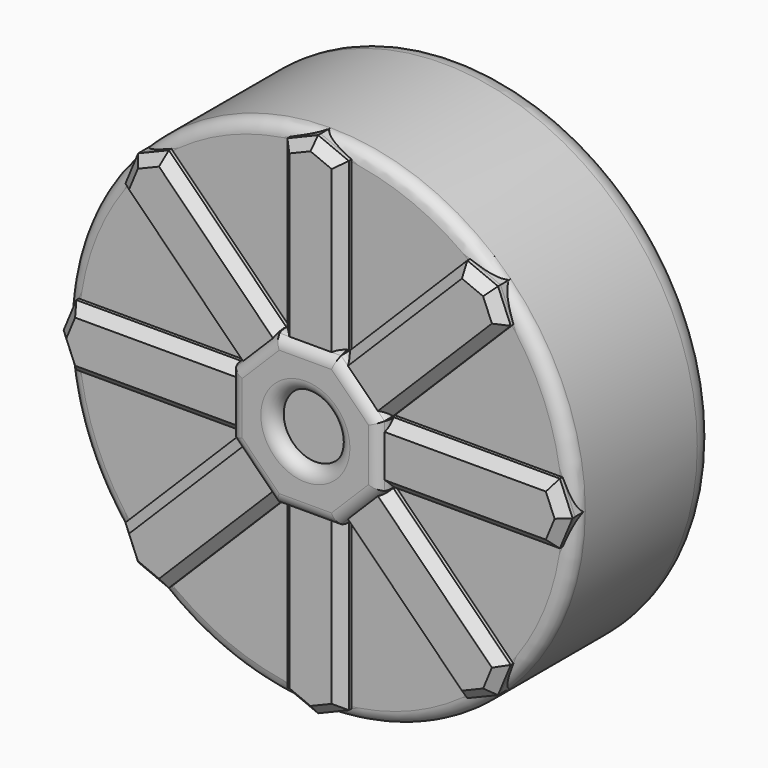
from build123d import *

# Parameters (mm, degrees)
F0_R           = 20
F1_DEPTH       = 14
F3_DEPTH       = 1
F5_DEPTH       = 0.5
F6_R           = 2.5
F7_DEPTH       = 1
F8_T4_ANGLE    = 45
F8_T9_ANGLE    = 45
F8_T15_ANGLE   = 45
F8_T20_ANGLE   = 45
F8_T26_ANGLE   = 45
F8_T31_ANGLE   = 45
F8_T37_ANGLE   = 45
F8_T42_ANGLE   = 45
F8_T48_ANGLE   = 45
F8_T53_ANGLE   = 45
F8_T59_ANGLE   = 45
F8_T64_ANGLE   = 45
F8_T70_ANGLE   = 45
F8_T75_ANGLE   = 45
F8_T81_ANGLE   = 45
F8_T86_ANGLE   = 45
F9_T1_DEPTH    = 9.1585541437
F9_T3_DEPTH    = 9.1585541437
F9_T5_DEPTH    = 9.1585541437
F9_T7_DEPTH    = 9.1585541437
F9_T9_DEPTH    = 9.1585541437
F9_T11_DEPTH   = 9.1585541437
F10_T1_DEPTH   = 6.4706504117
F10_T3_DEPTH   = 6.4706504117
F10_T5_DEPTH   = 6.4706504117
F10_T7_DEPTH   = 6.4706504117
F10_T9_DEPTH   = 6.4706504117
F10_T11_DEPTH  = 6.4706504117
F10_T13_DEPTH  = 6.4706504117
F10_T15_DEPTH  = 6.4706504117
F10_T17_DEPTH  = 6.4706504117
F10_T19_DEPTH  = 6.4706504117
F10_T21_DEPTH  = 6.4706504117
F10_T23_DEPTH  = 6.4706504117
F10_T25_DEPTH  = 6.4706504117
F10_T27_DEPTH  = 6.4706504117
F10_T29_DEPTH  = 6.4706504117
F10_T31_DEPTH  = 6.4706504117
F10_T36_DEPTH  = 17.0290973572
F10_S38_R      = 0.9999999996
F10_T39_DEPTH  = 10
F10_T43_DEPTH  = 17.0290973572
F10_S45_R      = 0.9999999996
F10_T46_DEPTH  = 10
F10_T50_DEPTH  = 17.0290973572
F10_S52_R      = 0.9999999996
F10_T53_DEPTH  = 10
F10_T57_DEPTH  = 17.0290973572
F10_S59_R      = 0.9999999996
F10_T60_DEPTH  = 10
F10_T64_DEPTH  = 17.0290973572
F10_S66_R      = 0.9999999996
F10_T67_DEPTH  = 10
F10_T71_DEPTH  = 17.0290973572
F10_S73_R      = 0.9999999996
F10_T74_DEPTH  = 10
F10_T78_DEPTH  = 17.0290973572
F10_S80_R      = 0.9999999996
F10_T81_DEPTH  = 10
F10_T85_DEPTH  = 17.0290973572
F10_S87_R      = 0.9999999996
F10_T88_DEPTH  = 10
F10_T92_DEPTH  = 17.0290973572
F10_S94_R      = 0.9999999996
F10_T95_DEPTH  = 10
F10_T99_DEPTH  = 17.0290973572
F10_S101_R     = 0.9999999996
F10_T102_DEPTH = 10
F10_T106_DEPTH = 17.0290973572
F10_S108_R     = 0.9999999996
F10_T109_DEPTH = 10
F10_T113_DEPTH = 17.0290973572
F10_S115_R     = 0.9999999996
F10_T116_DEPTH = 10
F10_T120_DEPTH = 17.0290973572
F10_S122_R     = 0.9999999996
F10_T123_DEPTH = 10
F10_T127_DEPTH = 17.0290973572
F10_S129_R     = 0.9999999996
F10_T130_DEPTH = 10
F10_T134_DEPTH = 17.0290973572
F10_S136_R     = 0.9999999996
F10_T137_DEPTH = 10
F10_T141_DEPTH = 17.0290973572
F10_S143_R     = 0.9999999996
F10_T144_DEPTH = 10
F11_R          = 2


# Not quite as in the source:
# - a fillet or chamfer that OpenCascade refuses, or shapes differently, is made with other operations: its cross-section is extruded or revolved along the edge and cut away or added


with BuildPart() as f1:
    # F0 (on Front) → F1 (new body)
    with BuildSketch(Plane.XZ):
        Circle(F0_R)
    extrude(amount=F1_DEPTH)

    # F2 (on face) → F3 (join)
    with BuildSketch(Plane.XZ.offset(14)):
        Polygon((15.1421356237, 11.7279220614), (14.1421356237, 14.1421356237), (11.7279220614, 15.1421356237), (2.4142135624, 5.8284271247), (2.4142135624, 19), (0, 20), (-2.4142135624, 19), (-2.4142135624, 5.8284271247), (-11.7279220614, 15.1421356237), (-14.1421356237, 14.1421356237), (-15.1421356237, 11.7279220614), (-5.8284271247, 2.4142135624), (-19, 2.4142135624), (-20, 0), (-19, -2.4142135624), (-5.8284271247, -2.4142135624), (-15.1421356237, -11.7279220614), (-14.1421356237, -14.1421356237), (-11.7279220614, -15.1421356237), (-2.4142135624, -5.8284271247), (-2.4142135624, -19), (0, -20), (2.4142135624, -19), (2.4142135624, -5.8284271247), (11.7279220614, -15.1421356237), (14.1421356237, -14.1421356237), (15.1421356237, -11.7279220614), (5.8284271247, -2.4142135624), (19, -2.4142135624), (20, 0), (19, 2.4142135624), (5.8284271247, 2.4142135624), align=None)
    extrude(amount=F3_DEPTH)

    # F4 (on face) → F5 (join)
    with BuildSketch(Plane.XZ.offset(15)):
        Polygon((2.4142135624, 5.8284271247), (-2.4142135624, 5.8284271247), (-5.8284271247, 2.4142135624), (-5.8284271247, -2.4142135624), (-2.4142135624, -5.8284271247), (2.4142135624, -5.8284271247), (5.8284271247, -2.4142135624), (5.8284271247, 2.4142135624), align=None)
    extrude(amount=F5_DEPTH)

    # F6 (on face) → F7 (cut)
    with BuildSketch(Plane.XZ.offset(15.5)):
        Circle(F6_R)
    extrude(amount=-F7_DEPTH, mode=Mode.SUBTRACT)

    # F8: fillet of radius 1 on 8 edges, made by hand


with BuildPart() as f8_tool2:
    # F8_s3 → F8_t4 (revolve)
    with BuildSketch(Plane(origin=(0, 0, 0), x_dir=(0, 1, 0), z_dir=(0.7071067812, 0, 0.7071067812))):
        with BuildLine():
            ThreePointArc((-13, 20), (-13.7071067812, 19.7071067812), (-14, 19))
            Line((-14, 19), (-14, 20))
            Line((-14, 20), (-13, 20))
        make_face()
    revolve(axis=Axis((0, -14, 0), (0, -1, 0)), revolution_arc=F8_T4_ANGLE)

    split(bisect_by=Plane(origin=(-17.0710678119, 0, 7.0710678119), x_dir=(0, 1, 0), z_dir=(-0.9238795325, 0, 0.3826834324)), keep=Keep.TOP)


with BuildPart() as f1_1:
    add(f1.part)

    # F8_t1: cut F8_tool2
    add(f8_tool2.part, mode=Mode.SUBTRACT)


with BuildPart() as f8_tool7:
    # F8_s8 → F8_t9 (revolve)
    with BuildSketch(Plane(origin=(0, 0, 0), x_dir=(0, 1, 0), z_dir=(0.7071067812, 0, 0.7071067812))):
        with BuildLine():
            ThreePointArc((-13, 20), (-13.7071067812, 19.7071067812), (-14, 19))
            Line((-14, 19), (-14, 20))
            Line((-14, 20), (-13, 20))
        make_face()
    revolve(axis=Axis((0, -14, 0), (0, -1, 0)), revolution_arc=F8_T9_ANGLE)

    split(bisect_by=Plane(origin=(-1.7071067812, 0, -1.7071067812), x_dir=(0, 1, 0), z_dir=(-0.7071067812, 0, -0.7071067812)), keep=Keep.TOP)

    split(bisect_by=Plane.XY.offset(2.4142135624), keep=Keep.TOP)


with BuildPart() as f1_2:
    add(f1_1.part)

    # F8_t6: cut F8_tool7
    add(f8_tool7.part, mode=Mode.SUBTRACT)


with BuildPart() as f8_tool13:
    # F8_s14 → F8_t15 (revolve)
    with BuildSketch(Plane.XY):
        with BuildLine():
            ThreePointArc((-20, -13), (-19.7071067812, -13.7071067812), (-19, -14))
            Line((-19, -14), (-20, -14))
            Line((-20, -14), (-20, -13))
        make_face()
    revolve(axis=Axis((0, -14, 0), (0, -1, 0)), revolution_arc=F8_T15_ANGLE)

    split(bisect_by=Plane(origin=(-17.0710678119, 0, -7.0710678119), x_dir=(0, 1, 0), z_dir=(-0.9238795325, 0, -0.3826834324)), keep=Keep.TOP)


with BuildPart() as f1_3:
    add(f1_2.part)

    # F8_t12: cut F8_tool13
    add(f8_tool13.part, mode=Mode.SUBTRACT)


with BuildPart() as f8_tool18:
    # F8_s19 → F8_t20 (revolve)
    with BuildSketch(Plane.XY):
        with BuildLine():
            ThreePointArc((-20, -13), (-19.7071067812, -13.7071067812), (-19, -14))
            Line((-19, -14), (-20, -14))
            Line((-20, -14), (-20, -13))
        make_face()
    revolve(axis=Axis((0, -14, 0), (0, -1, 0)), revolution_arc=F8_T20_ANGLE)

    split(bisect_by=Plane.XY.offset(-2.4142135624), keep=Keep.BOTTOM)

    split(bisect_by=Plane(origin=(-1.7071067812, 0, 1.7071067812), x_dir=(0, 1, 0), z_dir=(-0.7071067812, 0, 0.7071067812)), keep=Keep.TOP)


with BuildPart() as f1_4:
    add(f1_3.part)

    # F8_t17: cut F8_tool18
    add(f8_tool18.part, mode=Mode.SUBTRACT)


with BuildPart() as f8_tool24:
    # F8_s25 → F8_t26 (revolve)
    with BuildSketch(Plane.YZ):
        with BuildLine():
            ThreePointArc((-13, 20), (-13.7071067812, 19.7071067812), (-14, 19))
            Line((-14, 19), (-14, 20))
            Line((-14, 20), (-13, 20))
        make_face()
    revolve(axis=Axis((0, -14, 0), (0, -1, 0)), revolution_arc=F8_T26_ANGLE)

    split(bisect_by=Plane(origin=(-7.0710678119, 0, 17.0710678119), x_dir=(0, 1, 0), z_dir=(-0.3826834324, 0, 0.9238795325)), keep=Keep.TOP)


with BuildPart() as f1_5:
    add(f1_4.part)

    # F8_t23: cut F8_tool24
    add(f8_tool24.part, mode=Mode.SUBTRACT)


with BuildPart() as f8_tool29:
    # F8_s30 → F8_t31 (revolve)
    with BuildSketch(Plane.YZ):
        with BuildLine():
            ThreePointArc((-13, 20), (-13.7071067812, 19.7071067812), (-14, 19))
            Line((-14, 19), (-14, 20))
            Line((-14, 20), (-13, 20))
        make_face()
    revolve(axis=Axis((0, -14, 0), (0, -1, 0)), revolution_arc=F8_T31_ANGLE)

    split(bisect_by=Plane.YZ.offset(-2.4142135624), keep=Keep.BOTTOM)

    split(bisect_by=Plane(origin=(1.7071067812, 0, 1.7071067812), x_dir=(0, 1, 0), z_dir=(0.7071067812, 0, 0.7071067812)), keep=Keep.TOP)


with BuildPart() as f1_6:
    add(f1_5.part)

    # F8_t28: cut F8_tool29
    add(f8_tool29.part, mode=Mode.SUBTRACT)


with BuildPart() as f8_tool35:
    # F8_s36 → F8_t37 (revolve)
    with BuildSketch(Plane(origin=(0, 0, 0), x_dir=(0, 1, 0), z_dir=(0.7071067812, 0, -0.7071067812))):
        with BuildLine():
            ThreePointArc((-13, 20), (-13.7071067812, 19.7071067812), (-14, 19))
            Line((-14, 19), (-14, 20))
            Line((-14, 20), (-13, 20))
        make_face()
    revolve(axis=Axis((0, -14, 0), (0, -1, 0)), revolution_arc=F8_T37_ANGLE)

    split(bisect_by=Plane(origin=(7.0710678119, 0, 17.0710678119), x_dir=(0, 1, 0), z_dir=(0.3826834324, 0, 0.9238795325)), keep=Keep.TOP)


with BuildPart() as f1_7:
    add(f1_6.part)

    # F8_t34: cut F8_tool35
    add(f8_tool35.part, mode=Mode.SUBTRACT)


with BuildPart() as f8_tool40:
    # F8_s41 → F8_t42 (revolve)
    with BuildSketch(Plane(origin=(0, 0, 0), x_dir=(0, 1, 0), z_dir=(0.7071067812, 0, -0.7071067812))):
        with BuildLine():
            ThreePointArc((-13, 20), (-13.7071067812, 19.7071067812), (-14, 19))
            Line((-14, 19), (-14, 20))
            Line((-14, 20), (-13, 20))
        make_face()
    revolve(axis=Axis((0, -14, 0), (0, -1, 0)), revolution_arc=F8_T42_ANGLE)

    split(bisect_by=Plane(origin=(-1.7071067812, 0, 1.7071067812), x_dir=(0, 1, 0), z_dir=(-0.7071067812, 0, 0.7071067812)), keep=Keep.TOP)

    split(bisect_by=Plane.YZ.offset(2.4142135624), keep=Keep.TOP)


with BuildPart() as f1_8:
    add(f1_7.part)

    # F8_t39: cut F8_tool40
    add(f8_tool40.part, mode=Mode.SUBTRACT)


with BuildPart() as f8_tool46:
    # F8_s47 → F8_t48 (revolve)
    with BuildSketch(Plane.XY):
        with BuildLine():
            ThreePointArc((20, -13), (19.7071067812, -13.7071067812), (19, -14))
            Line((19, -14), (20, -14))
            Line((20, -14), (20, -13))
        make_face()
    revolve(axis=Axis((0, -14, 0), (0, -1, 0)), revolution_arc=F8_T48_ANGLE)

    split(bisect_by=Plane(origin=(17.0710678119, 0, 7.0710678119), x_dir=(0, 1, 0), z_dir=(0.9238795325, 0, 0.3826834324)), keep=Keep.TOP)


with BuildPart() as f1_9:
    add(f1_8.part)

    # F8_t45: cut F8_tool46
    add(f8_tool46.part, mode=Mode.SUBTRACT)


with BuildPart() as f8_tool51:
    # F8_s52 → F8_t53 (revolve)
    with BuildSketch(Plane.XY):
        with BuildLine():
            ThreePointArc((20, -13), (19.7071067812, -13.7071067812), (19, -14))
            Line((19, -14), (20, -14))
            Line((20, -14), (20, -13))
        make_face()
    revolve(axis=Axis((0, -14, 0), (0, -1, 0)), revolution_arc=F8_T53_ANGLE)

    split(bisect_by=Plane.XY.offset(2.4142135624), keep=Keep.TOP)

    split(bisect_by=Plane(origin=(1.7071067812, 0, -1.7071067812), x_dir=(0, 1, 0), z_dir=(0.7071067812, 0, -0.7071067812)), keep=Keep.TOP)


with BuildPart() as f1_10:
    add(f1_9.part)

    # F8_t50: cut F8_tool51
    add(f8_tool51.part, mode=Mode.SUBTRACT)


with BuildPart() as f8_tool57:
    # F8_s58 → F8_t59 (revolve)
    with BuildSketch(Plane(origin=(0, 0, 0), x_dir=(0, 1, 0), z_dir=(-0.7071067812, 0, -0.7071067812))):
        with BuildLine():
            ThreePointArc((-13, 20), (-13.7071067812, 19.7071067812), (-14, 19))
            Line((-14, 19), (-14, 20))
            Line((-14, 20), (-13, 20))
        make_face()
    revolve(axis=Axis((0, -14, 0), (0, -1, 0)), revolution_arc=F8_T59_ANGLE)

    split(bisect_by=Plane(origin=(17.0710678119, 0, -7.0710678119), x_dir=(0, 1, 0), z_dir=(0.9238795325, 0, -0.3826834324)), keep=Keep.TOP)


with BuildPart() as f1_11:
    add(f1_10.part)

    # F8_t56: cut F8_tool57
    add(f8_tool57.part, mode=Mode.SUBTRACT)


with BuildPart() as f8_tool62:
    # F8_s63 → F8_t64 (revolve)
    with BuildSketch(Plane(origin=(0, 0, 0), x_dir=(0, 1, 0), z_dir=(-0.7071067812, 0, -0.7071067812))):
        with BuildLine():
            ThreePointArc((-13, 20), (-13.7071067812, 19.7071067812), (-14, 19))
            Line((-14, 19), (-14, 20))
            Line((-14, 20), (-13, 20))
        make_face()
    revolve(axis=Axis((0, -14, 0), (0, -1, 0)), revolution_arc=F8_T64_ANGLE)

    split(bisect_by=Plane(origin=(1.7071067812, 0, 1.7071067812), x_dir=(0, 1, 0), z_dir=(0.7071067812, 0, 0.7071067812)), keep=Keep.TOP)

    split(bisect_by=Plane.XY.offset(-2.4142135624), keep=Keep.BOTTOM)


with BuildPart() as f1_12:
    add(f1_11.part)

    # F8_t61: cut F8_tool62
    add(f8_tool62.part, mode=Mode.SUBTRACT)


with BuildPart() as f8_tool68:
    # F8_s69 → F8_t70 (revolve)
    with BuildSketch(Plane.YZ):
        with BuildLine():
            ThreePointArc((-13, -20), (-13.7071067812, -19.7071067812), (-14, -19))
            Line((-14, -19), (-14, -20))
            Line((-14, -20), (-13, -20))
        make_face()
    revolve(axis=Axis((0, -14, 0), (0, -1, 0)), revolution_arc=F8_T70_ANGLE)

    split(bisect_by=Plane(origin=(7.0710678119, 0, -17.0710678119), x_dir=(0, 1, 0), z_dir=(0.3826834324, 0, -0.9238795325)), keep=Keep.TOP)


with BuildPart() as f1_13:
    add(f1_12.part)

    # F8_t67: cut F8_tool68
    add(f8_tool68.part, mode=Mode.SUBTRACT)


with BuildPart() as f8_tool73:
    # F8_s74 → F8_t75 (revolve)
    with BuildSketch(Plane.YZ):
        with BuildLine():
            ThreePointArc((-13, -20), (-13.7071067812, -19.7071067812), (-14, -19))
            Line((-14, -19), (-14, -20))
            Line((-14, -20), (-13, -20))
        make_face()
    revolve(axis=Axis((0, -14, 0), (0, -1, 0)), revolution_arc=F8_T75_ANGLE)

    split(bisect_by=Plane.YZ.offset(2.4142135624), keep=Keep.TOP)

    split(bisect_by=Plane(origin=(-1.7071067812, 0, -1.7071067812), x_dir=(0, 1, 0), z_dir=(-0.7071067812, 0, -0.7071067812)), keep=Keep.TOP)


with BuildPart() as f1_14:
    add(f1_13.part)

    # F8_t72: cut F8_tool73
    add(f8_tool73.part, mode=Mode.SUBTRACT)


with BuildPart() as f8_tool79:
    # F8_s80 → F8_t81 (revolve)
    with BuildSketch(Plane(origin=(0, 0, 0), x_dir=(0, 1, 0), z_dir=(-0.7071067812, 0, 0.7071067812))):
        with BuildLine():
            ThreePointArc((-13, 20), (-13.7071067812, 19.7071067812), (-14, 19))
            Line((-14, 19), (-14, 20))
            Line((-14, 20), (-13, 20))
        make_face()
    revolve(axis=Axis((0, -14, 0), (0, -1, 0)), revolution_arc=F8_T81_ANGLE)

    split(bisect_by=Plane(origin=(-7.0710678119, 0, -17.0710678119), x_dir=(0, 1, 0), z_dir=(-0.3826834324, 0, -0.9238795325)), keep=Keep.TOP)


with BuildPart() as f1_15:
    add(f1_14.part)

    # F8_t78: cut F8_tool79
    add(f8_tool79.part, mode=Mode.SUBTRACT)


with BuildPart() as f8_tool84:
    # F8_s85 → F8_t86 (revolve)
    with BuildSketch(Plane(origin=(0, 0, 0), x_dir=(0, 1, 0), z_dir=(-0.7071067812, 0, 0.7071067812))):
        with BuildLine():
            ThreePointArc((-13, 20), (-13.7071067812, 19.7071067812), (-14, 19))
            Line((-14, 19), (-14, 20))
            Line((-14, 20), (-13, 20))
        make_face()
    revolve(axis=Axis((0, -14, 0), (0, -1, 0)), revolution_arc=F8_T86_ANGLE)

    split(bisect_by=Plane(origin=(1.7071067812, 0, -1.7071067812), x_dir=(0, 1, 0), z_dir=(0.7071067812, 0, -0.7071067812)), keep=Keep.TOP)

    split(bisect_by=Plane.YZ.offset(-2.4142135624), keep=Keep.BOTTOM)


with BuildPart() as f1_16:
    add(f1_15.part)

    # F8_t83: cut F8_tool84
    add(f8_tool84.part, mode=Mode.SUBTRACT)

    # F9: fillet of radius 1 on 9 edges, made by hand

    # F9_s2 → F9_t1 (cut)
    with BuildSketch(Plane.YZ.offset(-4.5792770718)):
        with BuildLine():
            ThreePointArc((-15.5, 4.962401721), (-15.3660254038, 5.462401721), (-15, 5.8284271247))
            Line((-15, 5.8284271247), (-15.5, 5.8284271247))
            Line((-15.5, 5.8284271247), (-15.5, 4.962401721))
        make_face()
        with BuildLine():
            ThreePointArc((-15.5, -4.962401721), (-15.3660254038, -5.462401721), (-15, -5.8284271247))
            Line((-15, -5.8284271247), (-15.5, -5.8284271247))
            Line((-15.5, -5.8284271247), (-15.5, -4.962401721))
        make_face()
    extrude(amount=F9_T1_DEPTH, mode=Mode.SUBTRACT)

    # F9_s4 → F9_t3 (cut)
    with BuildSketch(Plane(origin=(3.2380378704, 0, -3.2380378704), x_dir=(0, 1, 0), z_dir=(-0.7071067812, 0, 0.7071067812))):
        with BuildLine():
            ThreePointArc((-15.5, -4.962401721), (-15.3660254038, -5.462401721), (-15, -5.8284271247))
            Line((-15, -5.8284271247), (-15.5, -5.8284271247))
            Line((-15.5, -5.8284271247), (-15.5, -4.962401721))
        make_face()
    extrude(amount=F9_T3_DEPTH, mode=Mode.SUBTRACT)

    # F9_s6 → F9_t5 (cut)
    with BuildSketch(Plane(origin=(3.2380378704, 0, 3.2380378704), x_dir=(0, 1, 0), z_dir=(-0.7071067812, 0, -0.7071067812))):
        with BuildLine():
            ThreePointArc((-15.5, -4.962401721), (-15.3660254038, -5.462401721), (-15, -5.8284271247))
            Line((-15, -5.8284271247), (-15.5, -5.8284271247))
            Line((-15.5, -5.8284271247), (-15.5, -4.962401721))
        make_face()
    extrude(amount=F9_T5_DEPTH, mode=Mode.SUBTRACT)

    # F9_s8 → F9_t7 (cut)
    with BuildSketch(Plane.XY.offset(-4.5792770718)):
        with BuildLine():
            ThreePointArc((5.8284271247, -15), (5.462401721, -15.3660254038), (4.962401721, -15.5))
            Line((4.962401721, -15.5), (5.8284271247, -15.5))
            Line((5.8284271247, -15.5), (5.8284271247, -15))
        make_face()
        with BuildLine():
            ThreePointArc((-4.962401721, -15.5), (-5.462401721, -15.3660254038), (-5.8284271247, -15))
            Line((-5.8284271247, -15), (-5.8284271247, -15.5))
            Line((-5.8284271247, -15.5), (-4.962401721, -15.5))
        make_face()
    extrude(amount=F9_T7_DEPTH, mode=Mode.SUBTRACT)

    # F9_s10 → F9_t9 (cut)
    with BuildSketch(Plane(origin=(-3.2380378704, 0, -3.2380378704), x_dir=(0, 1, 0), z_dir=(0.7071067812, 0, 0.7071067812))):
        with BuildLine():
            ThreePointArc((-15.5, -4.962401721), (-15.3660254038, -5.462401721), (-15, -5.8284271247))
            Line((-15, -5.8284271247), (-15.5, -5.8284271247))
            Line((-15.5, -5.8284271247), (-15.5, -4.962401721))
        make_face()
    extrude(amount=F9_T9_DEPTH, mode=Mode.SUBTRACT)

    # F9_s12 → F9_t11 (cut)
    with BuildSketch(Plane(origin=(-3.2380378704, 0, 3.2380378704), x_dir=(0, 1, 0), z_dir=(0.7071067812, 0, -0.7071067812))):
        with BuildLine():
            ThreePointArc((-15.5, -4.962401721), (-15.3660254038, -5.462401721), (-15, -5.8284271247))
            Line((-15, -5.8284271247), (-15.5, -5.8284271247))
            Line((-15.5, -5.8284271247), (-15.5, -4.962401721))
        make_face()
    extrude(amount=F9_T11_DEPTH, mode=Mode.SUBTRACT)

    # F9_s13 → F9_t14 (revolve, cut)
    with BuildSketch(Plane.XY):
        with BuildLine():
            ThreePointArc((3.5, -15.5), (2.7928932188, -15.2071067812), (2.5, -14.5))
            Line((2.5, -14.5), (2.5, -15.5))
            Line((2.5, -15.5), (3.5, -15.5))
        make_face()
    revolve(axis=Axis((0, -15.5, 0), (0, -1, 0)), mode=Mode.SUBTRACT)

    # F10: chamfer of 0.75 on 32 edges, made by hand

    # F10_s2 → F10_t1 (cut)
    with BuildSketch(Plane(origin=(8.8530117694, 0, 3.6670375427), x_dir=(0, 1, 0), z_dir=(-0.9238795325, 0, -0.3826834324))):
        Polygon((-14.25, -18.4775906502), (-15, -17.7275906502), (-15, -18.4775906502), align=None)
    extrude(amount=F10_T1_DEPTH, mode=Mode.SUBTRACT)

    # F10_s4 → F10_t3 (cut)
    with BuildSketch(Plane(origin=(-2.874910292, 0, 1.1908268335), x_dir=(0, 1, 0), z_dir=(-0.9238795325, 0, 0.3826834324))):
        Polygon((-14.25, -18.4775906502), (-15, -17.7275906502), (-15, -18.4775906502), align=None)
    extrude(amount=F10_T3_DEPTH, mode=Mode.SUBTRACT)

    # F10_s6 → F10_t5 (cut)
    with BuildSketch(Plane(origin=(8.8530117694, 0, -3.6670375427), x_dir=(0, 1, 0), z_dir=(-0.9238795325, 0, 0.3826834324))):
        Polygon((-14.25, -18.4775906502), (-15, -17.7275906502), (-15, -18.4775906502), align=None)
    extrude(amount=F10_T5_DEPTH, mode=Mode.SUBTRACT)

    # F10_s8 → F10_t7 (cut)
    with BuildSketch(Plane(origin=(-1.1908268335, 0, 2.874910292), x_dir=(0, 1, 0), z_dir=(-0.3826834324, 0, 0.9238795325))):
        Polygon((-14.25, -18.4775906502), (-15, -17.7275906502), (-15, -18.4775906502), align=None)
    extrude(amount=F10_T7_DEPTH, mode=Mode.SUBTRACT)

    # F10_s10 → F10_t9 (cut)
    with BuildSketch(Plane(origin=(3.6670375427, 0, -8.8530117694), x_dir=(0, 1, 0), z_dir=(-0.3826834324, 0, 0.9238795325))):
        Polygon((-14.25, -18.4775906502), (-15, -17.7275906502), (-15, -18.4775906502), align=None)
    extrude(amount=F10_T9_DEPTH, mode=Mode.SUBTRACT)

    # F10_s12 → F10_t11 (cut)
    with BuildSketch(Plane(origin=(1.1908268335, 0, 2.874910292), x_dir=(0, 1, 0), z_dir=(0.3826834324, 0, 0.9238795325))):
        Polygon((-14.25, -18.4775906502), (-15, -17.7275906502), (-15, -18.4775906502), align=None)
    extrude(amount=F10_T11_DEPTH, mode=Mode.SUBTRACT)

    # F10_s14 → F10_t13 (cut)
    with BuildSketch(Plane(origin=(-3.6670375427, 0, -8.8530117694), x_dir=(0, 1, 0), z_dir=(0.3826834324, 0, 0.9238795325))):
        Polygon((-14.25, -18.4775906502), (-15, -17.7275906502), (-15, -18.4775906502), align=None)
    extrude(amount=F10_T13_DEPTH, mode=Mode.SUBTRACT)

    # F10_s16 → F10_t15 (cut)
    with BuildSketch(Plane(origin=(2.874910292, 0, 1.1908268335), x_dir=(0, 1, 0), z_dir=(0.9238795325, 0, 0.3826834324))):
        Polygon((-14.25, -18.4775906502), (-15, -17.7275906502), (-15, -18.4775906502), align=None)
    extrude(amount=F10_T15_DEPTH, mode=Mode.SUBTRACT)

    # F10_s18 → F10_t17 (cut)
    with BuildSketch(Plane(origin=(-8.8530117694, 0, -3.6670375427), x_dir=(0, 1, 0), z_dir=(0.9238795325, 0, 0.3826834324))):
        Polygon((-14.25, -18.4775906502), (-15, -17.7275906502), (-15, -18.4775906502), align=None)
    extrude(amount=F10_T17_DEPTH, mode=Mode.SUBTRACT)

    # F10_s20 → F10_t19 (cut)
    with BuildSketch(Plane(origin=(2.874910292, 0, -1.1908268335), x_dir=(0, 1, 0), z_dir=(0.9238795325, 0, -0.3826834324))):
        Polygon((-14.25, -18.4775906502), (-15, -17.7275906502), (-15, -18.4775906502), align=None)
    extrude(amount=F10_T19_DEPTH, mode=Mode.SUBTRACT)

    # F10_s22 → F10_t21 (cut)
    with BuildSketch(Plane(origin=(-8.8530117694, 0, 3.6670375427), x_dir=(0, 1, 0), z_dir=(0.9238795325, 0, -0.3826834324))):
        Polygon((-14.25, -18.4775906502), (-15, -17.7275906502), (-15, -18.4775906502), align=None)
    extrude(amount=F10_T21_DEPTH, mode=Mode.SUBTRACT)

    # F10_s24 → F10_t23 (cut)
    with BuildSketch(Plane(origin=(1.1908268335, 0, -2.874910292), x_dir=(0, 1, 0), z_dir=(0.3826834324, 0, -0.9238795325))):
        Polygon((-14.25, -18.4775906502), (-15, -17.7275906502), (-15, -18.4775906502), align=None)
    extrude(amount=F10_T23_DEPTH, mode=Mode.SUBTRACT)

    # F10_s26 → F10_t25 (cut)
    with BuildSketch(Plane(origin=(-3.6670375427, 0, 8.8530117694), x_dir=(0, 1, 0), z_dir=(0.3826834324, 0, -0.9238795325))):
        Polygon((-14.25, -18.4775906502), (-15, -17.7275906502), (-15, -18.4775906502), align=None)
    extrude(amount=F10_T25_DEPTH, mode=Mode.SUBTRACT)

    # F10_s28 → F10_t27 (cut)
    with BuildSketch(Plane(origin=(-1.1908268335, 0, -2.874910292), x_dir=(0, 1, 0), z_dir=(-0.3826834324, 0, -0.9238795325))):
        Polygon((-14.25, -18.4775906502), (-15, -17.7275906502), (-15, -18.4775906502), align=None)
    extrude(amount=F10_T27_DEPTH, mode=Mode.SUBTRACT)

    # F10_s30 → F10_t29 (cut)
    with BuildSketch(Plane(origin=(3.6670375427, 0, 8.8530117694), x_dir=(0, 1, 0), z_dir=(-0.3826834324, 0, -0.9238795325))):
        Polygon((-14.25, -18.4775906502), (-15, -17.7275906502), (-15, -18.4775906502), align=None)
    extrude(amount=F10_T29_DEPTH, mode=Mode.SUBTRACT)

    # F10_s32 → F10_t31 (cut)
    with BuildSketch(Plane(origin=(-2.874910292, 0, -1.1908268335), x_dir=(0, 1, 0), z_dir=(-0.9238795325, 0, -0.3826834324))):
        Polygon((-14.25, -18.4775906502), (-15, -17.7275906502), (-15, -18.4775906502), align=None)
    extrude(amount=F10_T31_DEPTH, mode=Mode.SUBTRACT)


with BuildPart() as f10_tool34:
    # F10_s35 → F10_t36 (new body)
    with BuildSketch(Plane.XY.offset(20.928762241)):
        Polygon((-1.6642135624, -15), (-2.4142135624, -14.25), (-2.4142135624, -15), align=None)
    extrude(amount=-F10_T36_DEPTH)

    split(bisect_by=Plane(origin=(1.7071067812, 0, 1.7071067812), x_dir=(0, 1, 0), z_dir=(0.7071067812, 0, 0.7071067812)), keep=Keep.TOP)

    # F10_s38 → F10_t39 (cut, symmetric)
    with BuildSketch(Plane.YZ.offset(-2)):
        with Locations((-14.5000000004, 4.9624017211)):
            Circle(F10_S38_R)
    extrude(amount=F10_T39_DEPTH, both=True, mode=Mode.SUBTRACT)


with BuildPart() as f1_17:
    add(f1_16.part)

    # F10_t33: cut F10_tool34
    add(f10_tool34.part, mode=Mode.SUBTRACT)


with BuildPart() as f10_tool41:
    # F10_s42 → F10_t43 (new body)
    with BuildSketch(Plane.XY.offset(3.8996648838)):
        Polygon((1.6642135624, -15), (2.4142135624, -14.25), (2.4142135624, -15), align=None)
    extrude(amount=F10_T43_DEPTH)

    split(bisect_by=Plane(origin=(-1.7071067812, 0, 1.7071067812), x_dir=(0, 1, 0), z_dir=(-0.7071067812, 0, 0.7071067812)), keep=Keep.TOP)

    # F10_s45 → F10_t46 (cut, symmetric)
    with BuildSketch(Plane.YZ.offset(2)):
        with Locations((-14.5000000004, 4.9624017211)):
            Circle(F10_S45_R)
    extrude(amount=F10_T46_DEPTH, both=True, mode=Mode.SUBTRACT)


with BuildPart() as f1_18:
    add(f1_17.part)

    # F10_t40: cut F10_tool41
    add(f10_tool41.part, mode=Mode.SUBTRACT)


with BuildPart() as f10_tool48:
    # F10_s49 → F10_t50 (new body)
    with BuildSketch(Plane(origin=(14.7988697024, 0, 14.7988697024), x_dir=(0, 1, 0), z_dir=(-0.7071067812, 0, -0.7071067812))):
        Polygon((-15, -1.6642135624), (-14.25, -2.4142135624), (-15, -2.4142135624), align=None)
    extrude(amount=F10_T50_DEPTH)

    split(bisect_by=Plane.YZ.offset(2.4142135624), keep=Keep.TOP)

    # F10_s52 → F10_t53 (cut, symmetric)
    with BuildSketch(Plane(origin=(-1.4142135624, 0, 1.4142135624), x_dir=(0, 1, 0), z_dir=(0.7071067812, 0, -0.7071067812))):
        with Locations((-14.5000000004, 4.9624017211)):
            Circle(F10_S52_R)
    extrude(amount=F10_T53_DEPTH, both=True, mode=Mode.SUBTRACT)


with BuildPart() as f1_19:
    add(f1_18.part)

    # F10_t47: cut F10_tool48
    add(f10_tool48.part, mode=Mode.SUBTRACT)


with BuildPart() as f10_tool55:
    # F10_s56 → F10_t57 (new body)
    with BuildSketch(Plane(origin=(2.7574794837, 0, 2.7574794837), x_dir=(0, 1, 0), z_dir=(0.7071067812, 0, 0.7071067812))):
        Polygon((-15, -1.6642135624), (-14.25, -2.4142135624), (-15, -2.4142135624), align=None)
    extrude(amount=F10_T57_DEPTH)

    split(bisect_by=Plane.XY.offset(2.4142135624), keep=Keep.TOP)

    # F10_s59 → F10_t60 (cut, symmetric)
    with BuildSketch(Plane(origin=(1.4142135624, 0, -1.4142135624), x_dir=(0, 1, 0), z_dir=(0.7071067812, 0, -0.7071067812))):
        with Locations((-14.5000000004, 4.9624017211)):
            Circle(F10_S59_R)
    extrude(amount=F10_T60_DEPTH, both=True, mode=Mode.SUBTRACT)


with BuildPart() as f1_20:
    add(f1_19.part)

    # F10_t54: cut F10_tool55
    add(f10_tool55.part, mode=Mode.SUBTRACT)


with BuildPart() as f10_tool62:
    # F10_s63 → F10_t64 (new body)
    with BuildSketch(Plane.YZ.offset(20.928762241)):
        Polygon((-14.25, 2.4142135624), (-15, 1.6642135624), (-15, 2.4142135624), align=None)
    extrude(amount=-F10_T64_DEPTH)

    split(bisect_by=Plane(origin=(1.7071067812, 0, -1.7071067812), x_dir=(0, 1, 0), z_dir=(0.7071067812, 0, -0.7071067812)), keep=Keep.TOP)

    # F10_s66 → F10_t67 (cut, symmetric)
    with BuildSketch(Plane.XY.offset(2)):
        with Locations((4.9624017211, -14.5000000004)):
            Circle(F10_S66_R)
    extrude(amount=F10_T67_DEPTH, both=True, mode=Mode.SUBTRACT)


with BuildPart() as f1_21:
    add(f1_20.part)

    # F10_t61: cut F10_tool62
    add(f10_tool62.part, mode=Mode.SUBTRACT)


with BuildPart() as f10_tool69:
    # F10_s70 → F10_t71 (new body)
    with BuildSketch(Plane.YZ.offset(3.8996648838)):
        Polygon((-15, -1.6642135624), (-14.25, -2.4142135624), (-15, -2.4142135624), align=None)
    extrude(amount=F10_T71_DEPTH)

    split(bisect_by=Plane(origin=(1.7071067812, 0, 1.7071067812), x_dir=(0, 1, 0), z_dir=(0.7071067812, 0, 0.7071067812)), keep=Keep.TOP)

    # F10_s73 → F10_t74 (cut, symmetric)
    with BuildSketch(Plane.XY.offset(-2)):
        with Locations((4.9624017211, -14.5000000004)):
            Circle(F10_S73_R)
    extrude(amount=F10_T74_DEPTH, both=True, mode=Mode.SUBTRACT)


with BuildPart() as f1_22:
    add(f1_21.part)

    # F10_t68: cut F10_tool69
    add(f10_tool69.part, mode=Mode.SUBTRACT)


with BuildPart() as f10_tool76:
    # F10_s77 → F10_t78 (new body)
    with BuildSketch(Plane(origin=(14.7988697024, 0, -14.7988697024), x_dir=(0, 1, 0), z_dir=(-0.7071067812, 0, 0.7071067812))):
        Polygon((-15, -1.6642135624), (-14.25, -2.4142135624), (-15, -2.4142135624), align=None)
    extrude(amount=F10_T78_DEPTH)

    split(bisect_by=Plane.XY.offset(-2.4142135624), keep=Keep.BOTTOM)

    # F10_s80 → F10_t81 (cut, symmetric)
    with BuildSketch(Plane(origin=(1.4142135624, 0, 1.4142135624), x_dir=(0, 1, 0), z_dir=(-0.7071067812, 0, -0.7071067812))):
        with Locations((-14.5000000004, 4.9624017211)):
            Circle(F10_S80_R)
    extrude(amount=F10_T81_DEPTH, both=True, mode=Mode.SUBTRACT)


with BuildPart() as f1_23:
    add(f1_22.part)

    # F10_t75: cut F10_tool76
    add(f10_tool76.part, mode=Mode.SUBTRACT)


with BuildPart() as f10_tool83:
    # F10_s84 → F10_t85 (new body)
    with BuildSketch(Plane(origin=(2.7574794837, 0, -2.7574794837), x_dir=(0, 1, 0), z_dir=(0.7071067812, 0, -0.7071067812))):
        Polygon((-15, -1.6642135624), (-14.25, -2.4142135624), (-15, -2.4142135624), align=None)
    extrude(amount=F10_T85_DEPTH)

    split(bisect_by=Plane.YZ.offset(2.4142135624), keep=Keep.TOP)

    # F10_s87 → F10_t88 (cut, symmetric)
    with BuildSketch(Plane(origin=(-1.4142135624, 0, -1.4142135624), x_dir=(0, 1, 0), z_dir=(-0.7071067812, 0, -0.7071067812))):
        with Locations((-14.5000000004, 4.9624017211)):
            Circle(F10_S87_R)
    extrude(amount=F10_T88_DEPTH, both=True, mode=Mode.SUBTRACT)


with BuildPart() as f1_24:
    add(f1_23.part)

    # F10_t82: cut F10_tool83
    add(f10_tool83.part, mode=Mode.SUBTRACT)


with BuildPart() as f10_tool90:
    # F10_s91 → F10_t92 (new body)
    with BuildSketch(Plane.XY.offset(-20.928762241)):
        Polygon((1.6642135624, -15), (2.4142135624, -14.25), (2.4142135624, -15), align=None)
    extrude(amount=F10_T92_DEPTH)

    split(bisect_by=Plane(origin=(-1.7071067812, 0, -1.7071067812), x_dir=(0, 1, 0), z_dir=(-0.7071067812, 0, -0.7071067812)), keep=Keep.TOP)

    # F10_s94 → F10_t95 (cut, symmetric)
    with BuildSketch(Plane.YZ.offset(2)):
        with Locations((-14.5000000004, -4.9624017211)):
            Circle(F10_S94_R)
    extrude(amount=F10_T95_DEPTH, both=True, mode=Mode.SUBTRACT)


with BuildPart() as f1_25:
    add(f1_24.part)

    # F10_t89: cut F10_tool90
    add(f10_tool90.part, mode=Mode.SUBTRACT)


with BuildPart() as f10_tool97:
    # F10_s98 → F10_t99 (new body)
    with BuildSketch(Plane.XY.offset(-3.8996648838)):
        Polygon((-1.6642135624, -15), (-2.4142135624, -14.25), (-2.4142135624, -15), align=None)
    extrude(amount=-F10_T99_DEPTH)

    split(bisect_by=Plane(origin=(1.7071067812, 0, -1.7071067812), x_dir=(0, 1, 0), z_dir=(0.7071067812, 0, -0.7071067812)), keep=Keep.TOP)

    # F10_s101 → F10_t102 (cut, symmetric)
    with BuildSketch(Plane.YZ.offset(-2)):
        with Locations((-14.5000000004, -4.9624017211)):
            Circle(F10_S101_R)
    extrude(amount=F10_T102_DEPTH, both=True, mode=Mode.SUBTRACT)


with BuildPart() as f1_26:
    add(f1_25.part)

    # F10_t96: cut F10_tool97
    add(f10_tool97.part, mode=Mode.SUBTRACT)


with BuildPart() as f10_tool104:
    # F10_s105 → F10_t106 (new body)
    with BuildSketch(Plane(origin=(-14.7988697024, 0, -14.7988697024), x_dir=(0, 1, 0), z_dir=(0.7071067812, 0, 0.7071067812))):
        Polygon((-15, -1.6642135624), (-14.25, -2.4142135624), (-15, -2.4142135624), align=None)
    extrude(amount=F10_T106_DEPTH)

    split(bisect_by=Plane.YZ.offset(-2.4142135624), keep=Keep.BOTTOM)

    # F10_s108 → F10_t109 (cut, symmetric)
    with BuildSketch(Plane(origin=(1.4142135624, 0, -1.4142135624), x_dir=(0, 1, 0), z_dir=(-0.7071067812, 0, 0.7071067812))):
        with Locations((-14.5000000004, 4.9624017211)):
            Circle(F10_S108_R)
    extrude(amount=F10_T109_DEPTH, both=True, mode=Mode.SUBTRACT)


with BuildPart() as f1_27:
    add(f1_26.part)

    # F10_t103: cut F10_tool104
    add(f10_tool104.part, mode=Mode.SUBTRACT)


with BuildPart() as f10_tool111:
    # F10_s112 → F10_t113 (new body)
    with BuildSketch(Plane(origin=(-2.7574794837, 0, -2.7574794837), x_dir=(0, 1, 0), z_dir=(-0.7071067812, 0, -0.7071067812))):
        Polygon((-15, -1.6642135624), (-14.25, -2.4142135624), (-15, -2.4142135624), align=None)
    extrude(amount=F10_T113_DEPTH)

    split(bisect_by=Plane.XY.offset(-2.4142135624), keep=Keep.BOTTOM)

    # F10_s115 → F10_t116 (cut, symmetric)
    with BuildSketch(Plane(origin=(-1.4142135624, 0, 1.4142135624), x_dir=(0, 1, 0), z_dir=(-0.7071067812, 0, 0.7071067812))):
        with Locations((-14.5000000004, 4.9624017211)):
            Circle(F10_S115_R)
    extrude(amount=F10_T116_DEPTH, both=True, mode=Mode.SUBTRACT)


with BuildPart() as f1_28:
    add(f1_27.part)

    # F10_t110: cut F10_tool111
    add(f10_tool111.part, mode=Mode.SUBTRACT)


with BuildPart() as f10_tool118:
    # F10_s119 → F10_t120 (new body)
    with BuildSketch(Plane.YZ.offset(-20.928762241)):
        Polygon((-15, -1.6642135624), (-14.25, -2.4142135624), (-15, -2.4142135624), align=None)
    extrude(amount=F10_T120_DEPTH)

    split(bisect_by=Plane(origin=(-1.7071067812, 0, 1.7071067812), x_dir=(0, 1, 0), z_dir=(-0.7071067812, 0, 0.7071067812)), keep=Keep.TOP)

    # F10_s122 → F10_t123 (cut, symmetric)
    with BuildSketch(Plane.XY.offset(-2)):
        with Locations((-4.9624017211, -14.5000000004)):
            Circle(F10_S122_R)
    extrude(amount=F10_T123_DEPTH, both=True, mode=Mode.SUBTRACT)


with BuildPart() as f1_29:
    add(f1_28.part)

    # F10_t117: cut F10_tool118
    add(f10_tool118.part, mode=Mode.SUBTRACT)


with BuildPart() as f10_tool125:
    # F10_s126 → F10_t127 (new body)
    with BuildSketch(Plane.YZ.offset(-3.8996648838)):
        Polygon((-15, 1.6642135624), (-14.25, 2.4142135624), (-15, 2.4142135624), align=None)
    extrude(amount=-F10_T127_DEPTH)

    split(bisect_by=Plane(origin=(-1.7071067812, 0, -1.7071067812), x_dir=(0, 1, 0), z_dir=(-0.7071067812, 0, -0.7071067812)), keep=Keep.TOP)

    # F10_s129 → F10_t130 (cut, symmetric)
    with BuildSketch(Plane.XY.offset(2)):
        with Locations((-4.9624017211, -14.5000000004)):
            Circle(F10_S129_R)
    extrude(amount=F10_T130_DEPTH, both=True, mode=Mode.SUBTRACT)


with BuildPart() as f1_30:
    add(f1_29.part)

    # F10_t124: cut F10_tool125
    add(f10_tool125.part, mode=Mode.SUBTRACT)


with BuildPart() as f10_tool132:
    # F10_s133 → F10_t134 (new body)
    with BuildSketch(Plane(origin=(-14.7988697024, 0, 14.7988697024), x_dir=(0, 1, 0), z_dir=(0.7071067812, 0, -0.7071067812))):
        Polygon((-15, -1.6642135624), (-14.25, -2.4142135624), (-15, -2.4142135624), align=None)
    extrude(amount=F10_T134_DEPTH)

    split(bisect_by=Plane.XY.offset(2.4142135624), keep=Keep.TOP)

    # F10_s136 → F10_t137 (cut, symmetric)
    with BuildSketch(Plane(origin=(-1.4142135624, 0, -1.4142135624), x_dir=(0, 1, 0), z_dir=(0.7071067812, 0, 0.7071067812))):
        with Locations((-14.5000000004, 4.9624017211)):
            Circle(F10_S136_R)
    extrude(amount=F10_T137_DEPTH, both=True, mode=Mode.SUBTRACT)


with BuildPart() as f1_31:
    add(f1_30.part)

    # F10_t131: cut F10_tool132
    add(f10_tool132.part, mode=Mode.SUBTRACT)


with BuildPart() as f10_tool139:
    # F10_s140 → F10_t141 (new body)
    with BuildSketch(Plane(origin=(-2.7574794837, 0, 2.7574794837), x_dir=(0, 1, 0), z_dir=(-0.7071067812, 0, 0.7071067812))):
        Polygon((-15, -1.6642135624), (-14.25, -2.4142135624), (-15, -2.4142135624), align=None)
    extrude(amount=F10_T141_DEPTH)

    split(bisect_by=Plane.YZ.offset(-2.4142135624), keep=Keep.BOTTOM)

    # F10_s143 → F10_t144 (cut, symmetric)
    with BuildSketch(Plane(origin=(1.4142135624, 0, 1.4142135624), x_dir=(0, 1, 0), z_dir=(0.7071067812, 0, 0.7071067812))):
        with Locations((-14.5000000004, 4.9624017211)):
            Circle(F10_S143_R)
    extrude(amount=F10_T144_DEPTH, both=True, mode=Mode.SUBTRACT)


with BuildPart() as f1_32:
    add(f1_31.part)

    # F10_t138: cut F10_tool139
    add(f10_tool139.part, mode=Mode.SUBTRACT)

    # F11
    f11_edges = [f1_32.edges().sort_by_distance(p)[0] for p in [
        (-20, 0, 0),
    ]]
    fillet(f11_edges, radius=F11_R)


solid = f1_32.part
